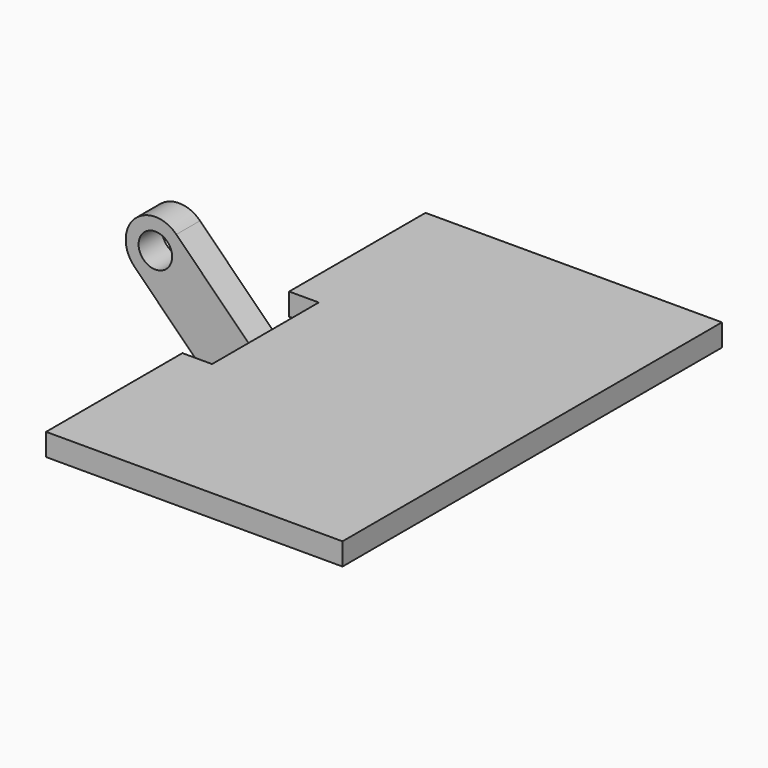
from build123d import *

# Parameters (mm, degrees)
F0_R      = 7.1882
F1_DEPTH  = 12.7
F2_START  = 12.7
F2_DEPTH  = 12.7
F3_R      = 12.69999
F3_2_R    = 12.69999
F5_START  = 25.4
F4_W      = 38.1
F4_H      = 25.4
F5_DEPTH  = 60.325
F6_DEPTH  = 19.05
F7_R      = 9.525
F8_DEPTH  = 25.4
F9_R      = 6.35
F10_DEPTH = 12.7
F12_DEPTH = 9.525
F13_DEPTH = 25.4


# Not quite as in the source:
# - a fillet or chamfer is up to 0.001 mm smaller than in the source, because OpenCascade refuses the exact size


with BuildPart() as f1:
    # F0 (on Front) → F1 (new body)
    with BuildSketch(Plane.XZ):
        Polygon((71.8420489686, -71.8420489686), (0, 0), (-17.9605122421, -17.9605122421), (53.8815367264, -89.8025612107), align=None)
        with Locations((0, -17.9605122421)):
            Circle(F0_R, mode=Mode.SUBTRACT)
        Polygon((89.8025612107, -89.8025612107), (71.8420489686, -71.8420489686), (53.8815367264, -89.8025612107), (71.8420489686, -107.7630734528), align=None)
        with Locations((71.8420489686, -89.8025612107)):
            Circle(F0_R, mode=Mode.SUBTRACT)
    extrude(amount=F1_DEPTH)

    # F3#2 (radius 12.7 in the source; OpenCascade refuses exactly that, so slightly less here)
    f3_2_edges = [f1.edges().sort_by_distance(p)[0] for p in [
        (89.802561, -6.35, -89.802561),
        (71.842049, -6.35, -107.763073),
        (0, -6.35, 0),
        (-17.960512, -6.35, -17.960512),
    ]]
    fillet(f3_2_edges, radius=F3_2_R)

    # F0 (on Front) → F6 (cut)
    with BuildSketch(Plane.XZ):
        with Locations((143.6840979371, -17.9605122421)):
            Circle(F0_R)
    extrude(amount=-F6_DEPTH, mode=Mode.SUBTRACT)


with BuildPart() as f2:
    # F0 (on Front) → F2 (new body)
    with BuildSketch(Plane.XZ.offset(F2_START)):
        Polygon((143.6840979371, 0), (71.8420489686, -71.8420489686), (89.8025612107, -89.8025612107), (161.6446101792, -17.9605122421), align=None)
        with Locations((143.6840979371, -17.9605122421)):
            Circle(F0_R, mode=Mode.SUBTRACT)
        Polygon((89.8025612107, -89.8025612107), (71.8420489686, -71.8420489686), (53.8815367264, -89.8025612107), (71.8420489686, -107.7630734528), align=None)
        with Locations((71.8420489686, -89.8025612107)):
            Circle(F0_R, mode=Mode.SUBTRACT)
    extrude(amount=F2_DEPTH)

    # F3 (radius 12.7 in the source; OpenCascade refuses exactly that, so slightly less here)
    f3_edges = [f2.edges().sort_by_distance(p)[0] for p in [
        (143.684098, -19.05, 0),
        (161.64461, -19.05, -17.960512),
        (53.881537, -19.05, -89.802561),
        (71.842049, -19.05, -107.763073),
    ]]
    fillet(f3_edges, radius=F3_R)

    # F4 (on face) → F5 (join)
    with BuildSketch(Plane.XZ.offset(F5_START)):
        with Locations((143.6840979371, -17.9605122421)):
            Rectangle(F4_W, F4_H)
    extrude(amount=F5_DEPTH)

    # F7 (on face) → F8 (cut)
    with BuildSketch(Plane.XY.offset(-5.2605122421)):
        with Locations((143.6840979371, -69.85)):
            Circle(F7_R)
    extrude(amount=-F8_DEPTH, mode=Mode.SUBTRACT)

    # F9 (on face) → F10 (cut)
    with BuildSketch(Plane(origin=(0, -25.4, 0), x_dir=(-1, 0, 0), z_dir=(0, 1, 0))):
        with Locations((-143.6840979371, -17.9605122421)):
            Circle(F9_R)
    extrude(amount=-F10_DEPTH, mode=Mode.SUBTRACT)


with BuildPart() as f12:
    # F11 (on face) → F12 (new body)
    with BuildSketch(Plane.XY.offset(-5.2605122421)):
        Polygon((80.1840979371, -98.425), (80.1840979371, -171.45), (207.1840979371, -171.45), (207.1840979371, 31.75), (80.1840979371, 31.75), (80.1840979371, -41.275), (92.8840979371, -41.275), (92.8840979371, -98.425), align=None)
    extrude(amount=F12_DEPTH)


with BuildPart() as f13:
    # F7 (on face) → F13 (new body)
    with BuildSketch(Plane.XY.offset(-5.2605122421)):
        with Locations((143.6840979371, -69.85)):
            Circle(F7_R)
    extrude(amount=-F13_DEPTH)


solid = Compound([f1.part, f2.part, f12.part, f13.part])
